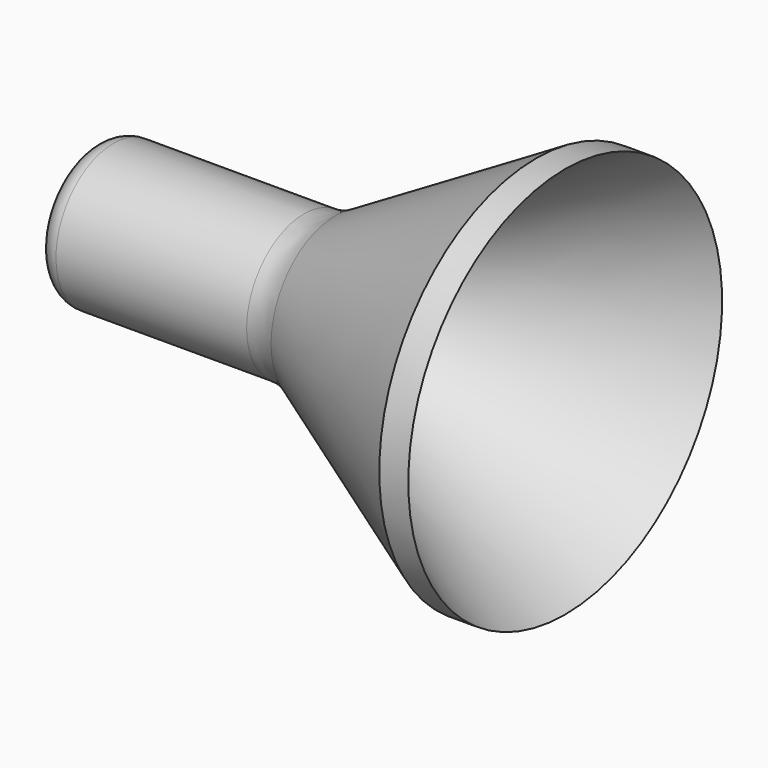
from build123d import *

# Parameters (mm, degrees)
F2_R = 4.99999
F3_R = 15


# Not quite as in the source:
# - a fillet or chamfer is up to 0.001 mm smaller than in the source, because OpenCascade refuses the exact size


with BuildPart() as f1:
    # F0 (on Front) → F1 (revolve)
    with BuildSketch(Plane.XZ):
        Polygon((55, 17.3), (0, 17.3), (0, 12.3), (55, 12.3), (113.9615242271, 47.3), (106.9615242271, 47.3), align=None)
    revolve(axis=Axis((19.2044641059, 0, 0), (1, 0, 0)))

    # F2 (radius 5 in the source; OpenCascade refuses exactly that, so slightly less here)
    f2_edges = [f1.edges().sort_by_distance(p)[0] for p in [
        (0, 0, -17.3),
    ]]
    fillet(f2_edges, radius=F2_R)

    # F3
    f3_edges = [f1.edges().sort_by_distance(p)[0] for p in [
        (55, 0, -17.3),
    ]]
    fillet(f3_edges, radius=F3_R)


solid = f1.part
